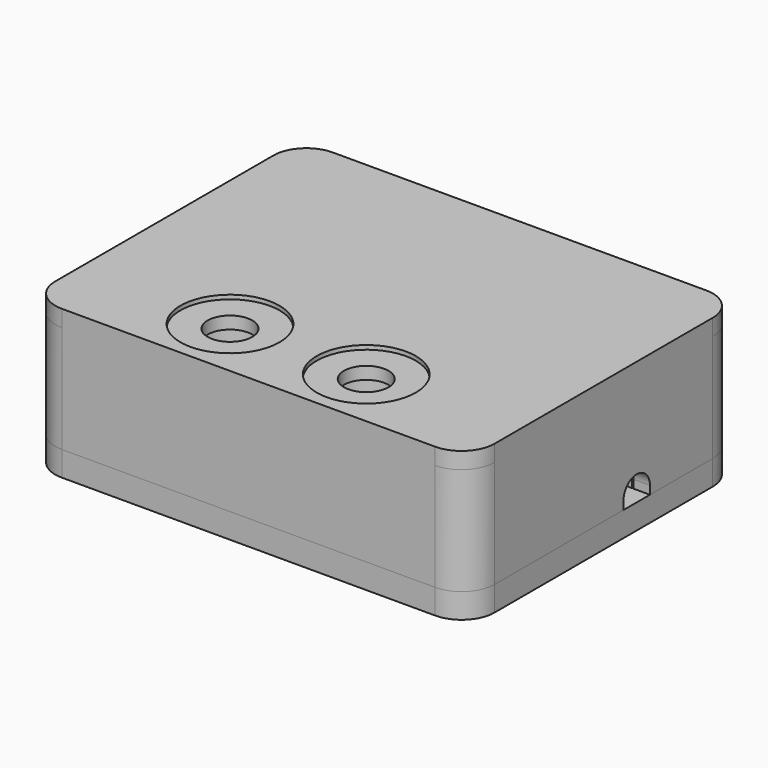
from build123d import *

# Parameters (mm, degrees)
F0_W      = 43.2
F0_H      = 21
F1_DEPTH  = 1.6
F2_R      = 0.75
F3_DEPTH  = 25
F4_W      = 7.5
F4_H      = 11
F5_DEPTH  = 10.5
F6_W      = 53.2
F6_H      = 41
F7_DEPTH  = 3
F8_R      = 2.7
F9_DEPTH  = 25
F10_W     = 53.2
F10_H     = 41
F10_W_2   = 49.2
F10_H_2   = 37
F11_DEPTH = 13
F12_R     = 2
F13_R     = 4
F13_2_R   = 4
F15_DEPTH = 2
F17_DEPTH = 2
F18_R     = 3.9
F18_R_2   = 2.7
F19_DEPTH = 10
F20_R     = 2.7
F21_DEPTH = 25
F22_R     = 5.3
F22_R_2   = 4.1
F23_DEPTH = 6
F25_DEPTH = 63.4
F26_R     = 6
F27_DEPTH = 0.5


with BuildPart() as f1:
    # F0 (on Top) → F1 (new body)
    with BuildSketch(Plane.XY):
        Rectangle(F0_W, F0_H)
    extrude(amount=F1_DEPTH)

    # F2 (on face) → F3 (cut)
    with BuildSketch(Plane.XY.offset(1.6)):
        with Locations((-19.25, 8.25)):
            Circle(F2_R)
        with Locations((-19.25, -8.25)):
            Circle(F2_R)
        with Locations((19.25, 8.25)):
            Circle(F2_R)
        with Locations((19.25, -8.25)):
            Circle(F2_R)
    extrude(amount=-F3_DEPTH, mode=Mode.SUBTRACT)

    # F4 (on face) → F5 (join)
    with BuildSketch(Plane.XY.offset(1.6)):
        with Locations((17.85, 0)):
            Rectangle(F4_W, F4_H)
        with Locations((-17.85, 0)):
            Rectangle(F4_W, F4_H)
    extrude(amount=F5_DEPTH)


with BuildPart() as f7:
    # F6 (on face) → F7 (new body)
    with BuildSketch(Plane(origin=(0, 0, 0), x_dir=(1, 0, 0), z_dir=(0, 0, -1))):
        with Locations((0, 5)):
            Rectangle(F6_W, F6_H)
    extrude(amount=F7_DEPTH)

    # F8 (on face) → F9 (cut)
    with BuildSketch(Plane.XY):
        with Locations((-8.25, -18)):
            Circle(F8_R)
        with Locations((8.25, -18)):
            Circle(F8_R)
    extrude(amount=-F9_DEPTH, mode=Mode.SUBTRACT)

    # F13
    f13_edges = [f7.edges().sort_by_distance(p)[0] for p in [
        (26.6, 15.5, -1.5),
        (-26.6, 15.5, -1.5),
        (-26.6, -25.5, -1.5),
        (26.6, -25.5, -1.5),
    ]]
    fillet(f13_edges, radius=F13_R)

    # F16 (on face) → F17 (join)
    with BuildSketch(Plane.XY):
        with BuildLine():
            Line((22.6, 13.3), (-22.6, 13.3))
            ThreePointArc((-22.6, 13.3), (-23.8727922061, 12.7727922061), (-24.4, 11.5))
            Line((-24.4, 11.5), (-24.4, -21.5))
            ThreePointArc((-24.4, -21.5), (-23.8727922061, -22.7727922061), (-22.6, -23.3))
            Line((-22.6, -23.3), (22.6, -23.3))
            ThreePointArc((22.6, -23.3), (23.8727922061, -22.7727922061), (24.4, -21.5))
            Line((24.4, -21.5), (24.4, 11.5))
            ThreePointArc((24.4, 11.5), (23.8727922061, 12.7727922061), (22.6, 13.3))
        make_face()
        with BuildLine():
            ThreePointArc((-23.4, 11.5), (-23.1656854249, 12.0656854249), (-22.6, 12.3))
            Line((-22.6, 12.3), (22.6, 12.3))
            ThreePointArc((22.6, 12.3), (23.1656854249, 12.0656854249), (23.4, 11.5))
            Line((23.4, 11.5), (23.4, -21.5))
            ThreePointArc((23.4, -21.5), (23.1656854249, -22.0656854249), (22.6, -22.3))
            Line((22.6, -22.3), (-22.6, -22.3))
            ThreePointArc((-22.6, -22.3), (-23.1656854249, -22.0656854249), (-23.4, -21.5))
            Line((-23.4, -21.5), (-23.4, 11.5))
        make_face(mode=Mode.SUBTRACT)
    extrude(amount=F17_DEPTH)

    # F18 (on face) → F19 (join)
    with BuildSketch(Plane.XY):
        with Locations((-8.25, -18)):
            Circle(F18_R)
        with Locations((-8.25, -18)):
            Circle(F18_R_2, mode=Mode.SUBTRACT)
        with Locations((8.25, -18)):
            Circle(F18_R)
        with Locations((8.25, -18)):
            Circle(F18_R_2, mode=Mode.SUBTRACT)
    extrude(amount=F19_DEPTH)


with BuildPart() as f11:
    # F10 (on face) → F11 (new body)
    with BuildSketch(Plane.XY):
        with Locations((0, -5)):
            Rectangle(F10_W, F10_H)
        with Locations((0, -5)):
            Rectangle(F10_W_2, F10_H_2, mode=Mode.SUBTRACT)
    extrude(amount=F11_DEPTH)

    # F12
    f12_edges = [f11.edges().sort_by_distance(p)[0] for p in [
        (24.6, 13.5, 6.5),
        (24.6, -23.5, 6.5),
        (-24.6, -23.5, 6.5),
        (-24.6, 13.5, 6.5),
    ]]
    fillet(f12_edges, radius=F12_R)

    # F13#2
    f13_2_edges = [f11.edges().sort_by_distance(p)[0] for p in [
        (26.6, 15.5, 6.5),
        (-26.6, 15.5, 6.5),
        (-26.6, -25.5, 6.5),
        (26.6, -25.5, 6.5),
    ]]
    fillet(f13_2_edges, radius=F13_2_R)

    # F14 (on face) → F15 (join)
    with BuildSketch(Plane.XY.offset(13)):
        with BuildLine():
            Line((-26.6, 11.5), (-26.6, -21.5))
            ThreePointArc((-26.6, -21.5), (-25.4284271247, -24.3284271247), (-22.6, -25.5))
            Line((-22.6, -25.5), (22.6, -25.5))
            ThreePointArc((22.6, -25.5), (25.4284271247, -24.3284271247), (26.6, -21.5))
            Line((26.6, -21.5), (26.6, 11.5))
            ThreePointArc((26.6, 11.5), (25.4284271247, 14.3284271247), (22.6, 15.5))
            Line((22.6, 15.5), (-22.6, 15.5))
            ThreePointArc((-22.6, 15.5), (-25.4284271247, 14.3284271247), (-26.6, 11.5))
        make_face()
    extrude(amount=F15_DEPTH)

    # F20 (on face) → F21 (cut)
    with BuildSketch(Plane.XY.offset(15)):
        with Locations((-8.25, -18)):
            Circle(F20_R)
        with Locations((8.25, -18)):
            Circle(F20_R)
    extrude(amount=-F21_DEPTH, mode=Mode.SUBTRACT)

    # F22 (on face) → F23 (join)
    with BuildSketch(Plane(origin=(0, 0, 13), x_dir=(1, 0, 0), z_dir=(0, 0, -1))):
        with Locations((-8.25, 18)):
            Circle(F22_R)
        with Locations((-8.25, 18)):
            Circle(F22_R_2, mode=Mode.SUBTRACT)
        with Locations((8.25, 18)):
            Circle(F22_R)
        with Locations((8.25, 18)):
            Circle(F22_R_2, mode=Mode.SUBTRACT)
    extrude(amount=F23_DEPTH)


with BuildPart() as f25_tool:
    # F24 (on face) → F25 (new body)
    with BuildSketch(Plane.YZ.offset(26.6)):
        with BuildLine():
            Line((-2, 1), (-2, 0))
            Line((-2, 0), (2, 0))
            Line((2, 0), (2, 1))
            ThreePointArc((2, 1), (1.4142135624, 2.4142135624), (0, 3))
            ThreePointArc((0, 3), (-1.4142135624, 2.4142135624), (-2, 1))
        make_face()
    extrude(amount=-F25_DEPTH)


with BuildPart() as f7_1:
    add(f7.part)

    # F25: cut by f25_tool
    add(f25_tool.part, mode=Mode.SUBTRACT)


with BuildPart() as f11_1:
    add(f11.part)

    # F25: cut by f25_tool
    add(f25_tool.part, mode=Mode.SUBTRACT)

    # F26 (on face) → F27 (cut)
    with BuildSketch(Plane.XY.offset(15)):
        with Locations((-8.25, -18)):
            Circle(F26_R)
        with Locations((8.25, -18)):
            Circle(F26_R)
    extrude(amount=-F27_DEPTH, mode=Mode.SUBTRACT)


solid = Compound([f1.part, f7_1.part, f11_1.part])
